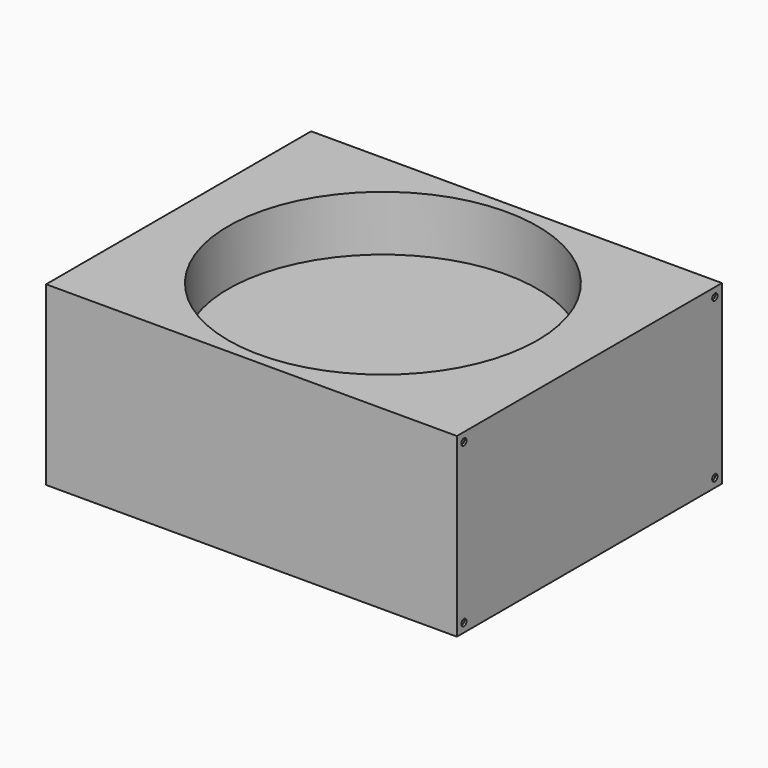
from build123d import *

# Parameters (mm, degrees)
F0_W         = 185
F0_H         = 150
F1_DEPTH     = 80
F2_R         = 70
F3_DEPTH     = 25
F5_TEXT_SIZE = 59.7476448036
F6_DEPTH     = 2
F4_R         = 1.5
F7_DEPTH     = 1
F9_W         = 6.2697291374
F9_H         = 11.2453848124
F9_W_2       = 40.1359349489
F9_W_3       = 23.6383453012
F9_W_4       = 22.2310088575
F9_W_5       = 28.1620938331
F9_W_6       = 27.9753450304
F9_W_7       = 22.9614675045
F9_W_8       = 16.0393565893
F9_W_9       = 13.9865353703
F9_W_10      = 15.0688141584
F9_W_11      = 21.7056125402
F10_DEPTH    = 2


# Not quite as in the source:
# - a feature names something its author has since deleted; it is built from what else it names
# - Text() gives the source's letters only with a copy of the font that has no kerning and outlines rounded to 1/6400 em; it was checked with that copy


with BuildPart() as f1:
    # F0 (on Top) → F1 (new body)
    with BuildSketch(Plane.XY):
        with Locations((-3500.6968264526, 75)):
            Rectangle(F0_W, F0_H)
    extrude(amount=F1_DEPTH)

    # F2 (on face) → F3 (cut)
    with BuildSketch(Plane.XY.offset(80)):
        with Locations((-3500.6968264526, 75)):
            Circle(F2_R)
    extrude(amount=-F3_DEPTH, mode=Mode.SUBTRACT)

    # F5 (on face) → F6 (join)
    with BuildSketch(Plane(origin=(0, 0, 0), x_dir=(1, 0, 0), z_dir=(0, 0, -1))):
        with Locations((-3548.8932132721, -75)):
            Text('Evga', F5_TEXT_SIZE, font='Open Sans', text_align=(TextAlign.LEFT, TextAlign.BOTTOM))
    extrude(amount=F6_DEPTH)

    # F4 (on face) → F7 (join)
    with BuildSketch(Plane.YZ.offset(-3408.1968264526)):
        Polygon((0, 6), (0, 0), (150, 0), (150, 80), (0, 80), align=None)
        with Locations((4, 4)):
            Circle(F4_R, mode=Mode.SUBTRACT)
        with Locations((146, 4)):
            Circle(F4_R, mode=Mode.SUBTRACT)
        Polygon((132, 35), (132, 33), (130, 35), align=None, mode=Mode.SUBTRACT)
        with Locations((4, 76)):
            Circle(F4_R, mode=Mode.SUBTRACT)
        with Locations((128.9848076105, 43.8655652106)):
            Circle(F4_R, mode=Mode.SUBTRACT)
        with Locations((146, 76)):
            Circle(F4_R, mode=Mode.SUBTRACT)
        with Locations((128.9848076105, 43.8655652106)):
            Circle(F4_R)
        Polygon((130, 35), (132, 33), (132, 35), align=None)
    extrude(amount=F7_DEPTH)

    # F9 (on face) → F10 (cut)
    with BuildSketch(Plane(origin=(-3593.1968264526, 0, 0), x_dir=(0, -1, 0), z_dir=(-1, 0, 0))):
        with Locations((-153.1348645687, 61.167344451)):
            Rectangle(F9_W, F9_H)
        with Locations((-108.1906631589, 61.167344451)):
            Rectangle(F9_W_2, F9_H)
        with Locations((-74.527297169, 61.167344451)):
            Rectangle(F9_W_3, F9_H)
        with Locations((-49.0837786347, 61.167344451)):
            Rectangle(F9_W_4, F9_H)
        with Locations((-22.1366016194, 61.167344451)):
            Rectangle(F9_W_5, F9_H)
        with Locations((-22.0432272181, 40.0260202587)):
            Rectangle(F9_W_6, F9_H)
        with Locations((-74.1888582706, 40.0260202587)):
            Rectangle(F9_W_7, F9_H)
        with Locations((-128.0083581805, 40.0260202587)):
            Rectangle(F9_W_8, F9_H)
        with Locations((-111.7168776691, 40.0260202587)):
            Rectangle(F9_W_9, F9_H)
        with Locations((-95.6571027637, 40.0260202587)):
            Rectangle(F9_W_10, F9_H)
        with Locations((-153.1348645687, 40.0260202587)):
            Rectangle(F9_W, F9_H)
        with Locations((-48.821080476, 40.0260202587)):
            Rectangle(F9_W_11, F9_H)
    extrude(amount=-F10_DEPTH, mode=Mode.SUBTRACT)


solid = f1.part
